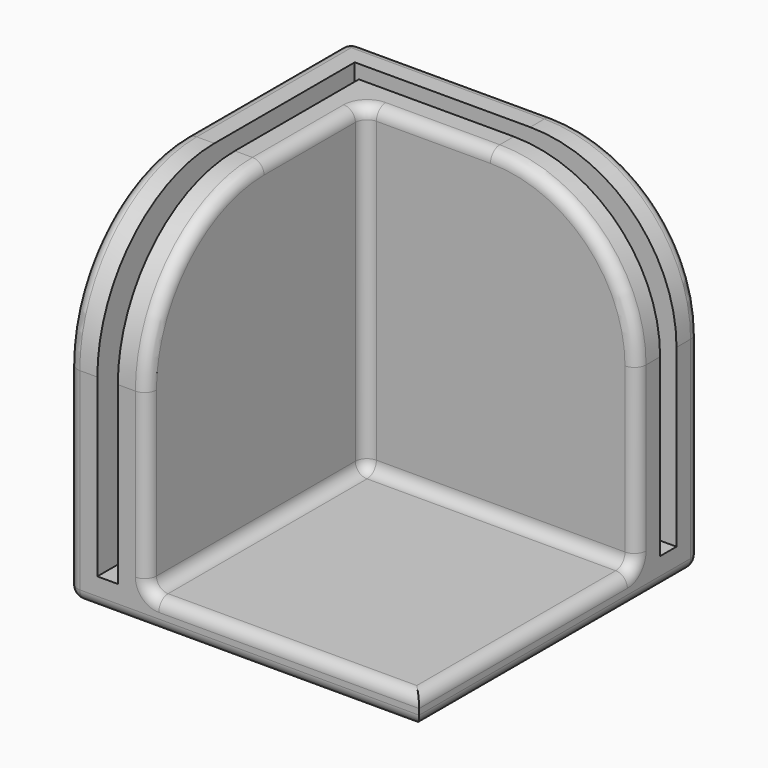
from build123d import *

# Parameters (mm, degrees)
F0_W     = 60
F0_H     = 60
F1_DEPTH = 5
F2_W     = 55
F2_H     = 5
F3_DEPTH = 55
F4_W     = 46.5
F4_H     = 5
F5_DEPTH = 55
F6_R     = 25
F7_R     = 2


with BuildPart() as f1:
    # F0 (on Top) → F1 (new body)
    with BuildSketch(Plane.XY):
        Rectangle(F0_W, F0_H)
    extrude(amount=F1_DEPTH)

    # F2 (on face) → F3 (join)
    with BuildSketch(Plane.XY.offset(5)):
        Polygon((-25, 30), (-30, 30), (-30, -30), (-25, -30), (-25, 25), align=None)
        with Locations((2.5, 27.5)):
            Rectangle(F2_W, F2_H)
    extrude(amount=F3_DEPTH)

    # F4 (on face) → F5 (join, through all)
    with BuildSketch(Plane.XY.offset(5)):
        Polygon((-21.5, 21.5), (-21.5, -30), (-16.5, -30), (-16.5, 16.5), (-16.5, 21.5), align=None)
        with Locations((6.75, 19)):
            Rectangle(F4_W, F4_H)
    extrude(amount=F5_DEPTH)

    # F6
    f6_edges = [f1.edges().sort_by_distance(p)[0] for p in [
        (-27.5, -30, 60),
        (-19, -30, 60),
        (30, 19, 60),
        (30, 27.5, 60),
    ]]
    fillet(f6_edges, radius=F6_R)

    # F7
    f7_edges = [f1.edges().sort_by_distance(p)[0] for p in [
        (30, 30, 17.5),
        (22.67767, 30, 52.67767),
        (0, 30, 0),
        (-12.5, 30, 60),
        (-30, 30, 30),
        (0, -30, 0),
        (30, 0, 0),
        (-30, 0, 0),
        (-30, 12.5, 60),
        (-30, -22.67767, 52.67767),
        (-30, -30, 17.5),
        (-16.5, -6.75, 5),
        (6.75, 16.5, 5),
        (30, -6.75, 5),
        (6.75, -30, 5),
        (-16.5, 16.5, 32.5),
        (-16.5, -30, 20),
        (30, 16.5, 20),
        (-16.5, -22.67767, 52.67767),
        (-16.5, 5.75, 60),
        (22.67767, 16.5, 52.67767),
        (-5.75, 16.5, 60),
    ]]
    fillet(f7_edges, radius=F7_R)


solid = f1.part
